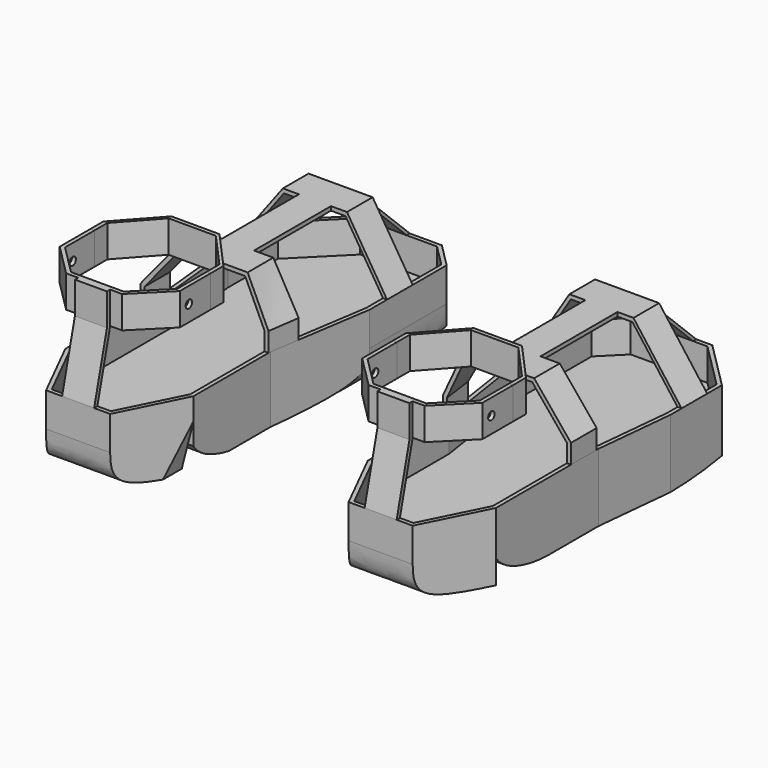
from build123d import *

# Parameters (mm, degrees)
F1_DEPTH       = 25.4
F5_DEPTH       = 12.7
F6_DEPTH       = 12.7
F8_DEPTH       = 25.4
F10_DEPTH      = 25.4
F12_DEPTH      = 3.175
F13_DEPTH      = 25.4
F15_DEPTH      = 19.05
F15_DEPTH_BACK = 6.35
F18_DEPTH      = 25.4
F20_DEPTH      = 25.4
F22_DEPTH      = 19.05
F22_DEPTH_BACK = 6.35
F23_DEPTH      = 6.35
F32_R          = 3.175
F33_DEPTH      = 114.301
F37_DEPTH      = 433.579
F39_DEPTH      = 304.8010001
F41_DEPTH      = 50.8


# Not quite as in the source:
# - a feature names something its author has since deleted; it is built from what else it names


with BuildPart() as f1:
    # F0 (on Top) → F1 (new body)
    with BuildSketch(Plane.XY):
        Polygon((3.175, 0), (0, 0), (0, -30.48), (25.4, -55.88), (69.85, -55.88), (95.25, -30.48), (95.25, 0), (92.075, 0), (92.075, -29.1648719395), (68.5348719395, -52.705), (26.7151280605, -52.705), (3.175, -29.1648719395), align=None)
    extrude(amount=-F1_DEPTH)

    # F4 (on offset) → F5 (join)
    with BuildSketch(Plane.YZ.offset(47.625)):
        Polygon((-68.58, -76.2), (-55.88, -25.4), (-55.88, 0), (-59.055, 0), (-59.055, -25.4), (-71.755, -76.2), (-71.755, -101.6), (-68.58, -101.6), align=None)
    extrude(amount=F5_DEPTH)

    # F6 (add): a face of the model
    f6_faces = [f1.faces().sort_by_distance(p)[0] for p in [
        (47.625, -63.8175, -50.8),
    ]]
    extrude(f6_faces, amount=F6_DEPTH)

    # F7 (on face) → F8 (join)
    with BuildSketch(Plane(origin=(0, 0, -101.6), x_dir=(1, 0, 0), z_dir=(0, 0, -1))):
        Polygon((34.925, 71.755), (22.225, 71.755), (-3.175, 20.955), (-3.175, -80.645), (-9.525, -144.145), (-9.525, -194.945), (28.575, -233.045), (92.075, -233.045), (111.125, -213.995), (111.125, -137.795), (98.425, -55.245), (98.425, 20.955), (73.025, 71.755), (60.325, 71.755), (60.325, 68.58), (71.0627420857, 68.58), (95.25, 20.2054841714), (95.25, -55.4878024703), (107.95, -138.0378024703), (107.95, -212.6798719395), (90.7598719395, -229.87), (29.8901280605, -229.87), (-6.35, -193.6298719395), (-6.35, -144.3033550971), (0, -80.8033550971), (0, 20.2054841714), (24.1872579143, 68.58), (34.925, 68.58), align=None)
    extrude(amount=-F8_DEPTH)

    # F11 (on face) → F12 (join)
    with BuildSketch(Plane(origin=(0, 0, -101.6), x_dir=(1, 0, 0), z_dir=(0, 0, -1))):
        Polygon((22.225, 71.755), (-3.175, 20.955), (-3.175, -80.645), (-9.525, -144.145), (-9.525, -194.945), (28.575, -233.045), (92.075, -233.045), (111.125, -213.995), (111.125, -137.795), (98.425, -55.245), (98.425, 20.955), (73.025, 71.755), align=None)
        Polygon((0, -80.8033550971), (0, 20.2054841714), (24.1872579143, 68.58), (71.0627420857, 68.58), (95.25, 20.2054841714), (95.25, -55.4878024703), (107.95, -138.0378024703), (107.95, -212.6798719395), (90.7598719395, -229.87), (29.8901280605, -229.87), (-6.35, -193.6298719395), (-6.35, -144.3033550971), align=None, mode=Mode.SUBTRACT)
        Polygon((24.1872579143, 68.58), (0, 20.2054841714), (0, -80.8033550971), (-6.35, -144.3033550971), (-6.35, -193.6298719395), (29.8901280605, -229.87), (90.7598719395, -229.87), (107.95, -212.6798719395), (107.95, -138.0378024703), (95.25, -55.4878024703), (95.25, 20.2054841714), (71.0627420857, 68.58), align=None)
    extrude(amount=F12_DEPTH)

    # F13 (add): a face of the model
    f13_faces = [f1.faces().sort_by_distance(p)[0] for p in [
        (50.1428916828, 88.9165130024, -104.775),
    ]]
    extrude(f13_faces, amount=F13_DEPTH)

    # F32 (on face) → F33 (cut, through all)
    with BuildSketch(Plane(origin=(-3.175, 0, 0), x_dir=(0, -1, 0), z_dir=(-1, 0, 0))):
        with Locations((21.59, -12.7)):
            Circle(F32_R)
    extrude(amount=-F33_DEPTH, mode=Mode.SUBTRACT)


with BuildPart() as f10:
    # F9 (on face) → F10 (new body)
    with BuildSketch(Plane.XY):
        Polygon((3.175, 12.7), (28.8925, 41.275), (66.3575, 41.275), (92.075, 12.7), (92.075, 0), (95.25, 0), (95.25, 12.7), (66.675, 44.45), (28.575, 44.45), (0, 12.7), (0, 0), (3.175, 0), align=None)
    extrude(amount=-F10_DEPTH)


with BuildPart() as f15:
    # F14 (on offset) → F15 (new body, two sides)
    with BuildSketch(Plane.YZ.offset(47.625)) as f15_sk:
        Polygon((180.34, -25.4), (59.69, -25.4), (59.69, -28.575), (180.4590625, -28.575), (229.87, -76.2), (233.045, -76.2), align=None)
    extrude(amount=F15_DEPTH)
    extrude(f15_sk.sketch, amount=-F15_DEPTH_BACK)

    # F17 (on plane+point) → F18 (join)
    with BuildSketch(Plane.XZ.offset(-180.34)):
        Polygon((41.275, -28.575), (41.275, -25.4), (28.575, -25.4), (-9.525, -76.2), (-6.35, -76.2), (29.36875, -28.575), align=None)
    extrude(amount=F18_DEPTH)

    # F19 (on plane+point) → F20 (join)
    with BuildSketch(Plane.XZ.offset(-180.34)):
        Polygon((79.375, -25.4), (66.675, -25.4), (66.675, -28.575), (78.184375, -28.575), (107.95, -76.2), (111.125, -76.2), align=None)
    extrude(amount=F20_DEPTH)

    # F21 (on face) → F22 (join, two sides)
    with BuildSketch(Plane.XZ.offset(-59.69)) as f22_sk:
        Polygon((-3.175, -76.2), (0, -76.2), (0, -62.0968352356), (27.5357932292, -28.575), (41.275, -28.575), (41.275, -25.4), (26.035, -25.4), (-3.175, -60.96), align=None)
    extrude(amount=-F22_DEPTH)
    extrude(f22_sk.sketch, amount=F22_DEPTH_BACK)

    # F23 (add, through all): a face of the model
    f23_faces = [f15.faces().sort_by_distance(p)[0] for p in [
        (53.975, 59.69, -26.9875),
    ]]
    extrude(f23_faces, amount=F23_DEPTH)

    # F24 (on face) → F29 section 0
    with BuildSketch(Plane.XZ.offset(-53.34)):
        Polygon((95.25, -76.2), (98.425, -76.2), (98.425, -60.96), (81.915, -25.4), (66.675, -25.4), (66.675, -28.575), (79.8885904855, -28.575), (95.25, -61.6611128005), align=None)
    # F28 (on plane+point) → F29 section 1
    with BuildSketch(Plane.XZ.offset(-78.74)):
        Polygon((98.8272611584, -76.2), (102.0396153846, -76.2), (102.0396153846, -60.96), (81.915, -25.4), (66.675, -25.4), (66.675, -28.575), (80.0636546231, -28.575), (98.8272611584, -61.730110577), align=None)
    loft()


with BuildPart() as f34_1:
    # F34: instance of F15
    add(f15.part.mirror(Plane.YZ.offset(167.513)))


with BuildPart() as f34_2:
    # F34: instance of F1
    add(f1.part.mirror(Plane.YZ.offset(167.513)))


with BuildPart() as f34_3:
    # F34: instance of F10
    add(f10.part.mirror(Plane.YZ.offset(167.513)))


with BuildPart() as f37_tool:
    # F36 (on offset) → F37 (new body, through all)
    with BuildSketch(Plane.YZ.offset(-89.027)):
        with BuildLine():
            Line((233.045, -130.175), (233.045, -103.1875))
            add(Edge.make_bspline(
                [(233.045, -103.1875), (233.045, -124.8658075929), (170.3352630138, -129.9640536308), (144.145, -130.175)],
                knots=[0, 0, 0, 0, 92.9060555413, 92.9060555413, 92.9060555413, 92.9060555413], degree=3))
            Line((144.145, -130.175), (194.945, -130.175))
            Line((194.945, -130.175), (233.045, -130.175))
        make_face()
        with BuildLine():
            Line((-71.755, -103.1875), (-71.755, -130.175))
            Line((-71.755, -130.175), (-20.955, -130.175))
            add(Edge.make_bspline(
                [(-20.955, -130.175), (-63.7144744396, -130.175), (-71.755, -127.5151520967), (-71.755, -103.1875)],
                knots=[0, 0, 0, 0, 57.5236052091, 57.5236052091, 57.5236052091, 57.5236052091], degree=3))
        make_face()
        with BuildLine():
            Line((-20.955, -111.125), (-20.955, -130.175))
            Line((-20.955, -130.175), (29.845, -130.175))
            add(Edge.make_bspline(
                [(29.845, -130.175), (13.0910566924, -129.8933892847), (-12.3976023346, -124.517044601), (-20.955, -111.125)],
                knots=[0, 0, 0, 0, 51.2531347773, 51.2531347773, 51.2531347773, 51.2531347773], degree=3))
        make_face()
    extrude(amount=F37_DEPTH)


with BuildPart() as f1_1:
    add(f1.part)

    # F37: cut by f37_tool
    add(f37_tool.part, mode=Mode.SUBTRACT)

    # F38 (on face) → F39 (cut, through all)
    with BuildSketch(Plane.XZ.offset(71.755)):
        with BuildLine():
            Line((-9.525, -130.175), (47.625, -130.175))
            add(Edge.make_bspline(
                [(47.625, -130.175), (-1.433890237, -130.175), (-8.6658653911, -127.8214102191), (-9.525, -115.4887963818)],
                knots=[0, 0, 0, 0, 49.7798205366, 49.7798205366, 49.7798205366, 49.7798205366], degree=3))
            Line((-9.525, -115.4887963818), (-9.525, -130.175))
        make_face()
        with BuildLine():
            add(Edge.make_bspline(
                [(80.687808733, -130.175), (108.4675369834, -129.6836903665), (111.125, -125.9703646635), (111.125, -103.1875)],
                knots=[16.1245146995, 16.1245146995, 16.1245146995, 16.1245146995, 68.9969213534, 68.9969213534, 68.9969213534, 68.9969213534], degree=3))
            Line((80.687808733, -130.175), (111.125, -130.175))
            Line((111.125, -130.175), (111.125, -103.1875))
        make_face()
    extrude(amount=-F39_DEPTH, mode=Mode.SUBTRACT)

    # F40 (on face) → F41 (cut, through all)
    with BuildSketch(Plane.XZ.offset(71.755)):
        Polygon((11.12416506, -129.1011813137), (-3.175, -93.6625), (-3.175, -129.8655213919), align=None)
        Polygon((98.425, -93.6625), (89.1219759688, -129.8655213919), (98.425, -129.8655213919), align=None)
    extrude(amount=-F41_DEPTH, mode=Mode.SUBTRACT)


with BuildPart() as f34_2_1:
    add(f34_2.part)

    # F37: cut by f37_tool
    add(f37_tool.part, mode=Mode.SUBTRACT)


solid = Compound([f10.part, f15.part, f34_1.part, f34_3.part, f1_1.part, f34_2_1.part])
